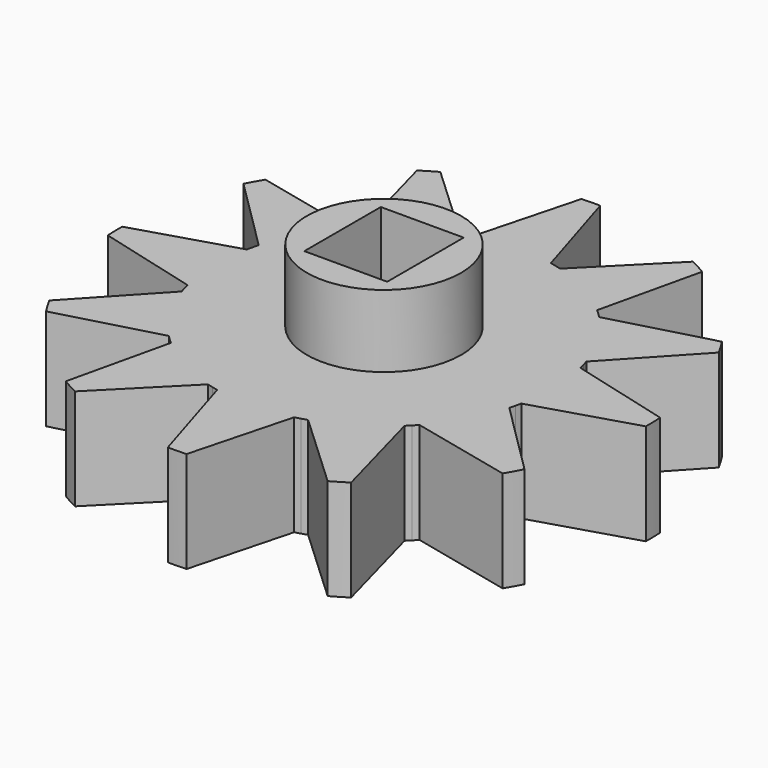
from build123d import *

# Parameters (mm, degrees)
F0_R            = 11
F1_DEPTH        = 4.2
F3_DEPTH        = 4.201
F3_COPIES_COUNT = 12
F5_R            = 3.2
F6_DEPTH        = 3
F7_W            = 3.4390550572
F7_H            = 3.9651677944
F8_DEPTH        = 7.201


# Not quite as in the source:
# - a pattern or mirror of a feature is missing from the dataset's text; its kind, count and spacing are read off the source's solid


with BuildPart() as f1:
    # F0 (on Top) → F1 (new body)
    with BuildSketch(Plane.XY):
        Circle(F0_R)
    extrude(amount=F1_DEPTH)

    # F2 (on face) → F3 (cut, through all)
    with BuildSketch(Plane(origin=(0, 0, 0), x_dir=(1, 0, 0), z_dir=(0, 0, -1))):
        with BuildLine():
            Line((-10.5683914605, 3.0510820928), (-6.7253400203, 1.9415976954))
            ThreePointArc((-6.7253400203, 1.9415976954), (-6.6904301664, 2.0586753481), (-6.6534823425, 2.1751259084))
            Line((-6.6534823425, 2.1751259084), (-9.6111801384, 5.3502538582))
            ThreePointArc((-9.6111801384, 5.3502538582), (-10.1550640166, 4.2278451744), (-10.5683914605, 3.0510820928))
        make_face()
        with BuildLine():
            ThreePointArc((-6.7890039073, 1.7057039447), (-6.7582012706, 1.8239286132), (-6.7253400203, 1.9415976954))
            Line((-6.7253400203, 1.9415976954), (-10.5683914605, 3.0510820928))
            ThreePointArc((-10.5683914605, 3.0510820928), (-10.8458486133, 1.8350934191), (-10.9838684057, 0.5955122546))
            Line((-10.9838684057, 0.5955122546), (-6.7890039073, 1.7057039447))
        make_face()
    f3 = extrude(amount=-F3_DEPTH, mode=Mode.SUBTRACT)

    # F3_copies: F3 ×12 about axis
    f3_copies_axis = Axis((0, 0, 0), (0, 0, 1))
    for i in range(1, F3_COPIES_COUNT):
        add(f3.rotate(f3_copies_axis, i * 360 / F3_COPIES_COUNT), mode=Mode.SUBTRACT)

    # F5 (on face) → F6 (join)
    with BuildSketch(Plane.XY.offset(4.2)):
        Circle(F5_R)
    extrude(amount=F6_DEPTH)

    # F7 (on face) → F8 (cut, through all)
    with BuildSketch(Plane.XY.offset(7.2)):
        Rectangle(F7_W, F7_H)
    extrude(amount=-F8_DEPTH, mode=Mode.SUBTRACT)


solid = f1.part
